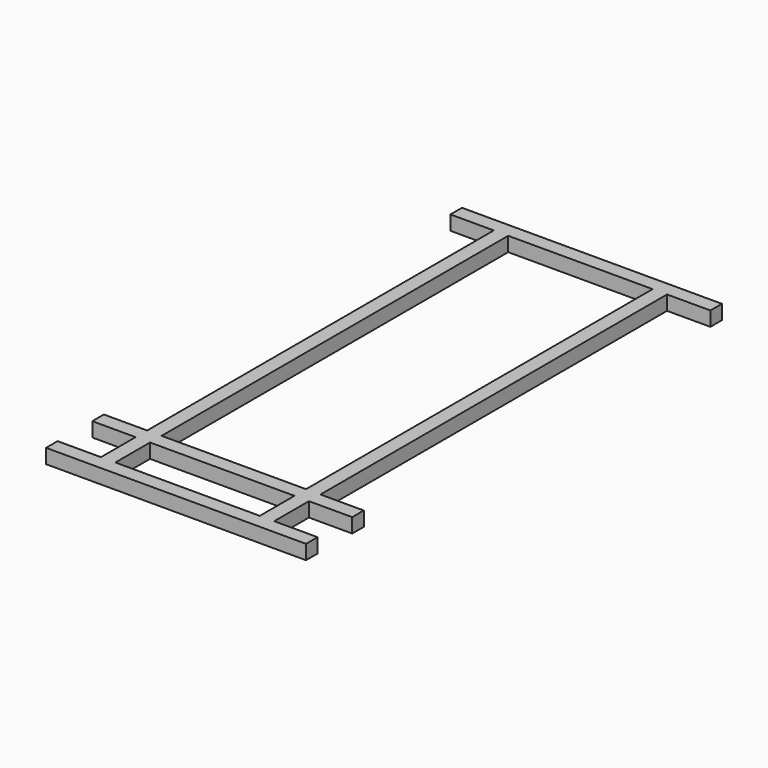
from build123d import *

# Parameters (mm, degrees)
F0_W     = 5.08
F0_H     = 5.08
F0_W_2   = 15.24
F0_W_3   = 50.8
F0_H_2   = 172.72
F1_DEPTH = 5.08
F2_W     = 5.08
F2_H     = 5.08
F3_DEPTH = 50.8
F4_W     = 5.08
F4_H     = 5.08
F5_DEPTH = 15.24
F6_W     = 5.08
F6_H     = 5.08
F7_DEPTH = 15.24


with BuildPart() as f1:
    # F0 (on Top) → F1 (new body)
    with BuildSketch(Plane.XY):
        with Locations((-74.2818623495, 91.6018860722)):
            Rectangle(F0_W, F0_H)
        with Locations((-84.4418623495, 91.6018860722)):
            Rectangle(F0_W_2, F0_H)
        with Locations((-46.3418623495, 91.6018860722)):
            Rectangle(F0_W_3, F0_H)
        with Locations((-74.2818623495, 2.7018860722)):
            Rectangle(F0_W, F0_H_2)
        with Locations((-18.4018623495, 91.6018860722)):
            Rectangle(F0_W, F0_H)
        with Locations((-74.2818623495, -86.1981139278)):
            Rectangle(F0_W, F0_H)
        with Locations((-84.4418623495, -86.1981139278)):
            Rectangle(F0_W_2, F0_H)
        with Locations((-46.3418623495, -86.1981139278)):
            Rectangle(F0_W_3, F0_H)
        with Locations((-18.4018623495, 2.7018860722)):
            Rectangle(F0_W, F0_H_2)
        with Locations((-8.2418623495, 91.6018860722)):
            Rectangle(F0_W_2, F0_H)
        with Locations((-18.4018623495, -86.1981139278)):
            Rectangle(F0_W, F0_H)
        with Locations((-8.2418623495, -86.1981139278)):
            Rectangle(F0_W_2, F0_H)
    extrude(amount=F1_DEPTH)

    # F2 (on face) → F3 (join)
    with BuildSketch(Plane.YZ.offset(-71.7418623495)):
        with Locations((-65.8781139278, 2.54)):
            Rectangle(F2_W, F2_H)
    extrude(amount=F3_DEPTH)

    # F4 (on face) → F5 (join)
    with BuildSketch(Plane.YZ.offset(-15.8618623495)):
        with Locations((-65.8781139278, 2.54)):
            Rectangle(F4_W, F4_H)
    extrude(amount=F5_DEPTH)

    # F6 (on face) → F7 (join)
    with BuildSketch(Plane(origin=(-76.8218623495, 0, 0), x_dir=(0, -1, 0), z_dir=(-1, 0, 0))):
        with Locations((65.8781139278, 2.54)):
            Rectangle(F6_W, F6_H)
    extrude(amount=F7_DEPTH)


solid = f1.part
